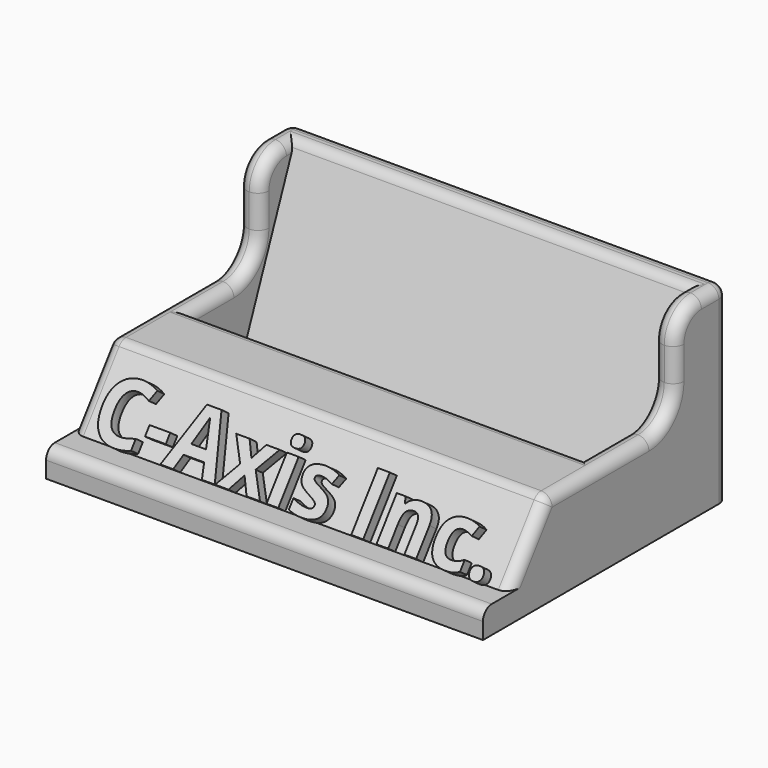
from build123d import *

# Parameters (mm, degrees)
F0_W           = 101.6
F0_H           = 71.12
F1_DEPTH       = 6.35
F2_W           = 101.6
F2_H           = 63.5
F3_DEPTH       = 38.1
F5_DEPTH       = 101.601
F6_TEXT_SIZE   = 18.3444444444
F7_DEPTH       = 2.54
F9_DEPTH       = 45.72
F9_DEPTH_BACK  = 45.72
F10_W          = 101.6
F10_H          = 22.86
F11_DEPTH      = 20.32
F11_DEPTH_BACK = 25.4
F12_R          = 7.62
F13_R          = 2.53999


# Not quite as in the source:
# - a fillet or chamfer is up to 0.001 mm smaller than in the source, because OpenCascade refuses the exact size
# - Text() gives the source's letters only with a copy of the font that has no kerning and outlines rounded to 1/6400 em; it was checked with that copy


with BuildPart() as f1:
    # F0 (on Top) → F1 (new body)
    with BuildSketch(Plane.XY):
        Rectangle(F0_W, F0_H)
    extrude(amount=F1_DEPTH)

    # F2 (on face) → F3 (join)
    with BuildSketch(Plane.XY.offset(6.35)):
        with Locations((0, 3.81)):
            Rectangle(F2_W, F2_H)
    extrude(amount=F3_DEPTH)

    # F4 (on face) → F5 (cut, through all)
    with BuildSketch(Plane.YZ.offset(50.8)):
        Polygon((-27.94, 44.45), (-27.94, 6.35), (0, 44.45), align=None)
    extrude(amount=-F5_DEPTH, mode=Mode.SUBTRACT)

    # F6 (on face) → F7 (join)
    with BuildSketch(Plane(origin=(0, -21.1972543353, 15.5446531792), x_dir=(1, 0, 0), z_dir=(0, -0.8064049959, 0.5913636636))):
        with Locations((-46.2800347222, -11.4020290381)):
            Text('C-Axis Inc.', F6_TEXT_SIZE, font='Open Sans', font_style=FontStyle.BOLD, text_align=(TextAlign.LEFT, TextAlign.BOTTOM))
    extrude(amount=F7_DEPTH)

    # F8 (on Right) → F9 (cut, two sides)
    with BuildSketch(Plane.YZ) as f9_sk:
        Polygon((-5.08, 6.35), (15.24, 6.35), (30.48, 44.45), (10.16, 44.45), align=None)
    extrude(amount=-F9_DEPTH, mode=Mode.SUBTRACT)
    extrude(f9_sk.sketch, amount=F9_DEPTH_BACK, mode=Mode.SUBTRACT)

    # F10 (on Front) → F11 (cut, two sides)
    with BuildSketch(Plane.XZ) as f11_sk:
        with Locations((0, 33.02)):
            Rectangle(F10_W, F10_H)
    extrude(amount=-F11_DEPTH, mode=Mode.SUBTRACT)
    extrude(f11_sk.sketch, amount=F11_DEPTH_BACK, mode=Mode.SUBTRACT)

    # F12
    f12_edges = [f1.edges().sort_by_distance(p)[0] for p in [
        (48.26, 20.32, 21.59),
        (-48.26, 20.32, 21.59),
        (48.26, 20.32, 44.45),
        (-48.26, 20.32, 44.45),
    ]]
    fillet(f12_edges, radius=F12_R)

    # F13 (radius 2.54 in the source; OpenCascade refuses exactly that, so slightly less here)
    f13_edges = [f1.edges().sort_by_distance(p)[0] for p in [
        (50.8, -2.032, 21.59),
        (45.72, 6.858, 21.59),
        (0, -35.56, 6.35),
        (-50.8, -22.352, 13.97),
        (50.8, -22.352, 13.97),
        (-50.8, -2.032, 21.59),
        (-45.72, 6.858, 21.59),
        (-50.8, 35.56, 22.225),
        (50.8, 35.56, 22.225),
        (0, 35.56, 44.45),
        (0, 30.48, 44.45),
        (0, -16.764, 21.59),
        (0, 1.016, 21.59),
    ]]
    fillet(f13_edges, radius=F13_R)


solid = f1.part
